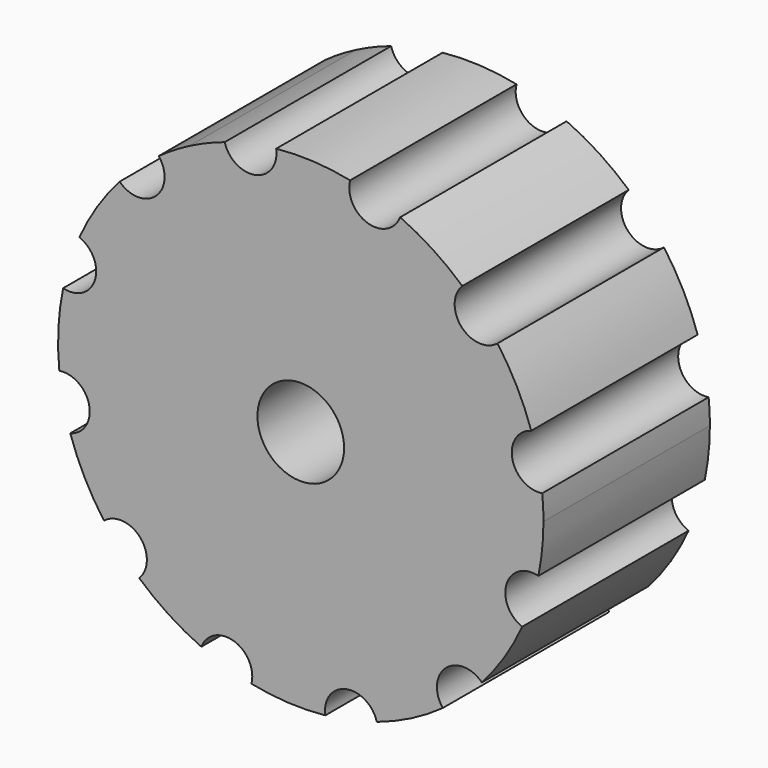
from build123d import *

# Parameters (mm, degrees)
F1_DEPTH = 12
F3_DEPTH = 25
F5_D     = 5


with BuildPart() as f1:
    # F0 (on Front) → F1 (new body)
    with BuildSketch(Plane.XZ):
        with BuildLine():
            ThreePointArc((-6.1837801054, 11.6114190374), (-6.2418651063, 12.0437074429), (-6.411999761, 12.4453308138))
            ThreePointArc((-6.411999761, 12.4453308138), (-7.8214415512, 11.6114190374), (-9.1238598826, 10.6186242444))
            ThreePointArc((-9.1238598826, 10.6186242444), (-7.2975070499, 10.0598302873), (-6.1837801054, 11.6114190374))
        make_face()
        with BuildLine():
            ThreePointArc((-9.1238598826, 10.6186242444), (-5.8423437781, -12.7226970088), (14, 0))
            ThreePointArc((14, 0), (7.2880725623, 11.9534094854), (-6.411999761, 12.4453308138))
            ThreePointArc((-6.411999761, 12.4453308138), (-6.2418651063, 12.0437074429), (-6.1837801054, 11.6114190374))
            ThreePointArc((-6.1837801054, 11.6114190374), (-7.2975070499, 10.0598302873), (-9.1238598826, 10.6186242444))
        make_face()
    extrude(amount=F1_DEPTH)

    # F2 (on face) → F3 (cut)
    with BuildSketch(Plane.XZ.offset(12)):
        with BuildLine():
            ThreePointArc((-10.4471785382, 9.3196813567), (-8.7916106337, 8.9938043215), (-7.8551114747, 10.3973962329))
            ThreePointArc((-7.8551114747, 10.3973962329), (-7.9419845398, 10.903914247), (-8.1926740651, 11.3525367942))
            ThreePointArc((-8.1926740651, 11.3525367942), (-9.3751880821, 10.3973962329), (-10.4471785382, 9.3196813567))
        make_face()
        with BuildLine():
            ThreePointArc((-10.4471785382, 9.3196813567), (-9.3751880821, 10.3973962329), (-8.1926740651, 11.3525367942))
            ThreePointArc((-8.1926740651, 11.3525367942), (-10.393116946, 11.5263132895), (-10.4471785382, 9.3196813567))
        make_face()
        with BuildLine():
            ThreePointArc((-1.4187954682, 13.9279222937), (-2.9204529279, 13.692003312), (-4.3876813336, 13.2946700792))
            ThreePointArc((-4.3876813336, 13.2946700792), (-2.720036717, 12.1851966772), (-1.4003763205, 13.692003312))
            ThreePointArc((-1.4003763205, 13.692003312), (-1.4049881033, 13.810321771), (-1.4187954682, 13.9279222937))
        make_face()
        with BuildLine():
            ThreePointArc((-1.4187954682, 13.9279222937), (-3.237546655, 15.1786385936), (-4.3876813336, 13.2946700792))
            ThreePointArc((-4.3876813336, 13.2946700792), (-2.9204529279, 13.692003312), (-1.4187954682, 13.9279222937))
        make_face()
        with BuildLine():
            ThreePointArc((-13.7073626903, 2.847491541), (-13.3178491608, 4.3168152299), (-12.7713322624, 5.7352482286))
            ThreePointArc((-12.7713322624, 5.7352482286), (-14.7638599444, 4.7855216477), (-13.7073626903, 2.847491541))
        make_face()
        with BuildLine():
            ThreePointArc((-11.7977725535, 4.3168152299), (-12.0645773537, 5.1770144334), (-12.7713322624, 5.7352482286))
            ThreePointArc((-12.7713322624, 5.7352482286), (-13.3178491608, 4.3168152299), (-13.7073626903, 2.847491541))
            ThreePointArc((-13.7073626903, 2.847491541), (-12.3908803135, 3.112090511), (-11.7977725535, 4.3168152299))
        make_face()
        with BuildLine():
            ThreePointArc((5.7352482286, 12.7713322624), (4.3168152299, 13.3178491608), (2.847491541, 13.7073626903))
            ThreePointArc((2.847491541, 13.7073626903), (3.8481088121, 11.8718383773), (5.7352482286, 12.7713322624))
        make_face()
        with BuildLine():
            ThreePointArc((5.8368918373, 13.3178491608), (4.5132182902, 14.825184137), (2.847491541, 13.7073626903))
            ThreePointArc((2.847491541, 13.7073626903), (4.3168152299, 13.3178491608), (5.7352482286, 12.7713322624))
            ThreePointArc((5.7352482286, 12.7713322624), (5.8112649134, 13.0399048573), (5.8368918373, 13.3178491608))
        make_face()
        with BuildLine():
            ThreePointArc((-12.1719267046, -2.9204529279), (-12.7040716425, -1.7651936891), (-13.9279222937, -1.4187954682))
            ThreePointArc((-13.9279222937, -1.4187954682), (-13.692003312, -2.9204529279), (-13.2946700792, -4.3876813336))
            ThreePointArc((-13.2946700792, -4.3876813336), (-12.4848144608, -3.8442104556), (-12.1719267046, -2.9204529279))
        make_face()
        with BuildLine():
            ThreePointArc((11.3525367942, 8.1926740651), (10.3973962329, 9.3751880821), (9.3196813567, 10.4471785382))
            ThreePointArc((9.3196813567, 10.4471785382), (9.2684791764, 8.3572592183), (11.3525367942, 8.1926740651))
        make_face()
        with BuildLine():
            ThreePointArc((11.9174728403, 9.3751880821), (10.9772340204, 10.7803290119), (9.3196813567, 10.4471785382))
            ThreePointArc((9.3196813567, 10.4471785382), (10.3973962329, 9.3751880821), (11.3525367942, 8.1926740651))
            ThreePointArc((11.3525367942, 8.1926740651), (11.7689864991, 8.719922461), (11.9174728403, 9.3751880821))
        make_face()
        with BuildLine():
            ThreePointArc((-8.8773196255, -9.3751880821), (-9.7421306118, -8.003597816), (-11.3525367942, -8.1926740651))
            ThreePointArc((-11.3525367942, -8.1926740651), (-10.3973962329, -9.3751880821), (-9.3196813567, -10.4471785382))
            ThreePointArc((-9.3196813567, -10.4471785382), (-8.9922553032, -9.9550258696), (-8.8773196255, -9.3751880821))
        make_face()
        with BuildLine():
            ThreePointArc((13.9279222937, 1.4187954682), (13.692003312, 2.9204529279), (13.2946700792, 4.3876813336))
            ThreePointArc((13.2946700792, 4.3876813336), (12.2053680304, 2.6033592009), (13.9279222937, 1.4187954682))
        make_face()
        with BuildLine():
            ThreePointArc((15.2120799194, 2.9204529279), (14.6157608397, 4.1276417791), (13.2946700792, 4.3876813336))
            ThreePointArc((13.2946700792, 4.3876813336), (13.692003312, 2.9204529279), (13.9279222937, 1.4187954682))
            ThreePointArc((13.9279222937, 1.4187954682), (14.8472625508, 1.9325212585), (15.2120799194, 2.9204529279))
        make_face()
        with BuildLine():
            ThreePointArc((-2.7967386225, -13.3178491608), (-4.0388709263, -11.8233994774), (-5.7352482286, -12.7713322624))
            ThreePointArc((-5.7352482286, -12.7713322624), (-4.3168152299, -13.3178491608), (-2.847491541, -13.7073626903))
            ThreePointArc((-2.847491541, -13.7073626903), (-2.8094802537, -13.5142522211), (-2.7967386225, -13.3178491608))
        make_face()
        with BuildLine():
            ThreePointArc((4.3876813336, -13.2946700792), (2.9204529279, -13.692003312), (1.4187954682, -13.9279222937))
            ThreePointArc((1.4187954682, -13.9279222937), (3.0387713869, -15.2074681366), (4.4405295353, -13.692003312))
            ThreePointArc((4.4405295353, -13.692003312), (4.4272595627, -13.4915871011), (4.3876813336, -13.2946700792))
        make_face()
        with BuildLine():
            ThreePointArc((4.3876813336, -13.2946700792), (2.6033592009, -12.2053680304), (1.4187954682, -13.9279222937))
            ThreePointArc((1.4187954682, -13.9279222937), (2.9204529279, -13.692003312), (4.3876813336, -13.2946700792))
        make_face()
        with BuildLine():
            ThreePointArc((12.7713322624, -5.7352482286), (13.3178491608, -4.3168152299), (13.7073626903, -2.847491541))
            ThreePointArc((13.7073626903, -2.847491541), (11.8718383773, -3.8481088121), (12.7713322624, -5.7352482286))
        make_face()
        with BuildLine():
            ThreePointArc((14.8379257682, -4.3168152299), (14.5225738798, -3.3898463825), (13.7073626903, -2.847491541))
            ThreePointArc((13.7073626903, -2.847491541), (13.3178491608, -4.3168152299), (12.7713322624, -5.7352482286))
            ThreePointArc((12.7713322624, -5.7352482286), (14.1780483644, -5.570087037), (14.8379257682, -4.3168152299))
        make_face()
        with BuildLine():
            ThreePointArc((10.4471785382, -9.3196813567), (8.3572592183, -9.2684791764), (8.1926740651, -11.3525367942))
            ThreePointArc((8.1926740651, -11.3525367942), (9.3751880821, -10.3973962329), (10.4471785382, -9.3196813567))
        make_face()
    extrude(amount=-F3_DEPTH, mode=Mode.SUBTRACT)

    # F5 (through all)
    with Locations(Plane(origin=(0, 0, 0), x_dir=(-1, 0, 0), z_dir=(0, 1, 0))):
        with Locations((0, 0)):
            Hole(F5_D / 2)


solid = f1.part
